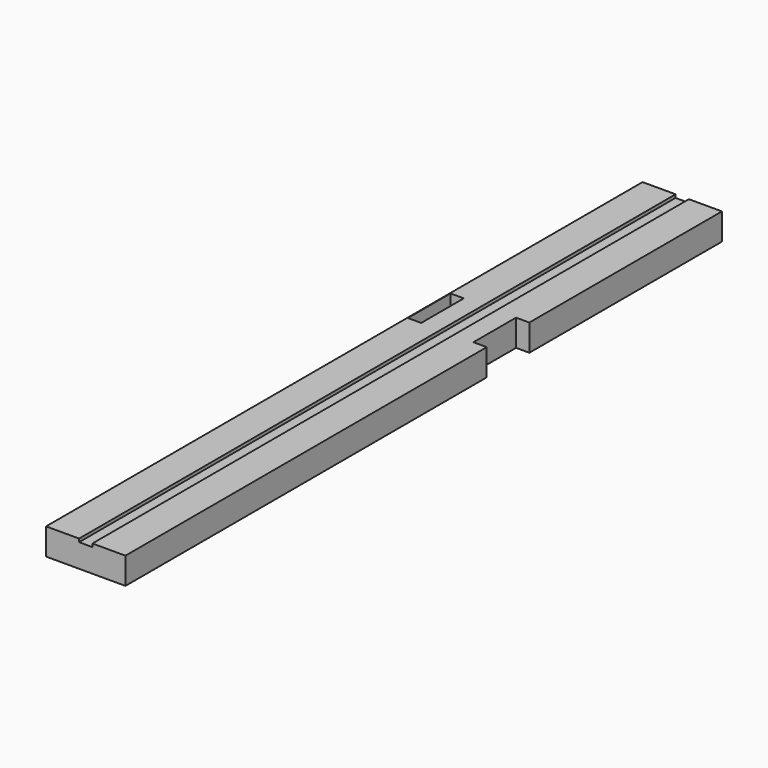
from build123d import *

# Parameters (mm, degrees)
F1_DEPTH = 355.6
F2_W     = 25.4
F2_H     = 12.7
F3_DEPTH = 6.35


# Not quite as in the source:
# - a pattern or mirror of a feature is missing from the dataset's text; its kind, count and spacing are read off the source's solid


with BuildPart() as f1:
    # F0 (on Front) → F1 (new body)
    with BuildSketch(Plane.XZ):
        Polygon((15.748, 12.7), (0, 12.7), (0, 0), (37.846, 0), (37.846, 12.7), (22.098, 12.7), (22.098, 11.176), (15.748, 11.176), align=None)
    extrude(amount=F1_DEPTH)

    # F2 (on face) → F3 (cut)
    with BuildSketch(Plane.YZ.offset(37.846)):
        with Locations((-127.508, 6.35)):
            Rectangle(F2_W, F2_H)
    f3 = extrude(amount=-F3_DEPTH, mode=Mode.SUBTRACT)

    # F3_copies: F3 across plane
    add(f3.mirror(Plane(origin=(19.05, 0, 0), x_dir=(0, 0, -1), z_dir=(-1, 0, 0))), mode=Mode.SUBTRACT)


solid = f1.part
